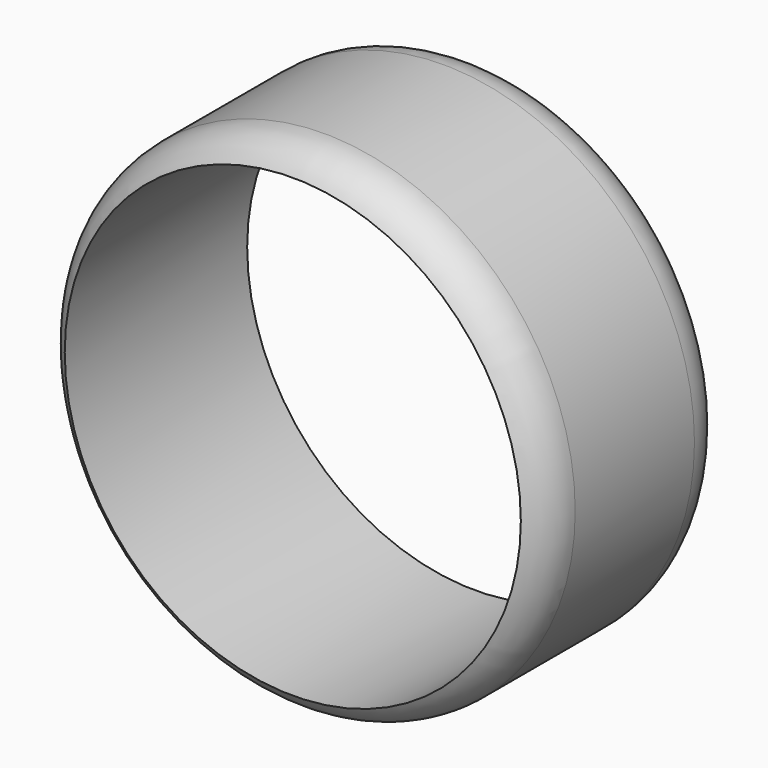
from build123d import *

# Parameters (mm, degrees)
F0_R     = 27.94
F0_R_2   = 25.4
F1_DEPTH = 25.4


# Not quite as in the source:
# - a fillet or chamfer that OpenCascade refuses, or shapes differently, is made with other operations: its cross-section is extruded or revolved along the edge and cut away or added


with BuildPart() as f1:
    # F0 (on Front) → F1 (new body)
    with BuildSketch(Plane.XZ):
        Circle(F0_R)
        Circle(F0_R_2, mode=Mode.SUBTRACT)
    extrude(amount=F1_DEPTH)

    # F2: fillet of radius 5.08 on 2 edges, made by hand

    # F2_s1 → F2_t2 (revolve, cut)
    with BuildSketch(Plane.XY):
        with BuildLine():
            ThreePointArc((27.94, -4.3994090512), (27.2594090512, -1.8594090512), (25.4, 0))
            Line((25.4, 0), (27.94, 0))
            Line((27.94, 0), (27.94, -4.3994090512))
        make_face()
    revolve(axis=Axis((0, 0, 0), (0, -1, 0)), mode=Mode.SUBTRACT)

    # F2_s3 → F2_t4 (revolve, cut)
    with BuildSketch(Plane.XY):
        with BuildLine():
            ThreePointArc((27.94, -21.0005909488), (27.2594090512, -23.5405909488), (25.4, -25.4))
            Line((25.4, -25.4), (27.94, -25.4))
            Line((27.94, -25.4), (27.94, -21.0005909488))
        make_face()
    revolve(axis=Axis((0, -25.4, 0), (0, -1, 0)), mode=Mode.SUBTRACT)


solid = f1.part
